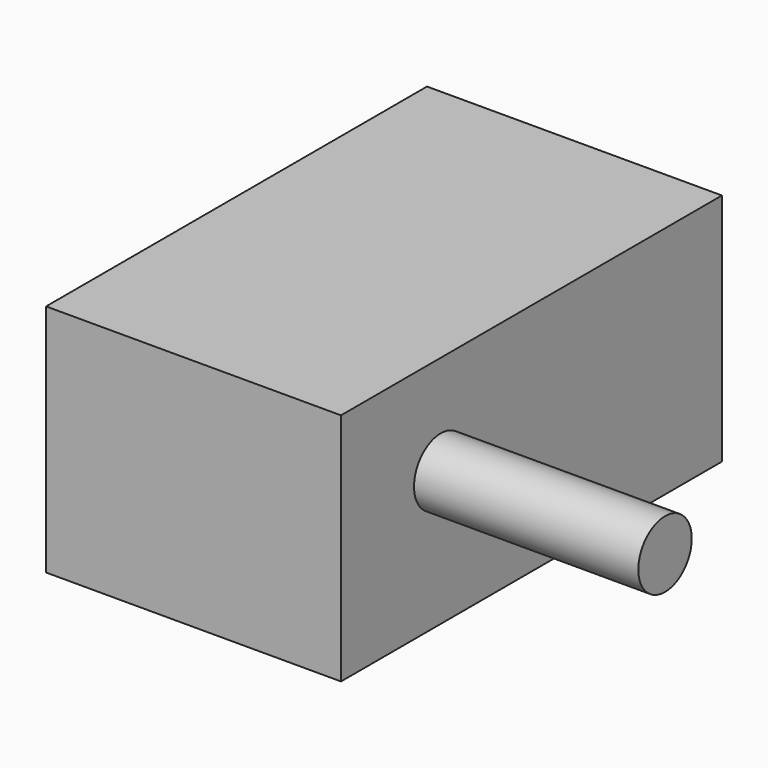
from build123d import *

# Parameters (mm, degrees)
F0_W     = 66.2436261773
F0_H     = 52.6286661625
F1_DEPTH = 53.9066623896
F2_DEPTH = 53.045405075
F3_R     = 7.4993670996
F4_DEPTH = 84.1025914997


# Not quite as in the source:
# - a feature names something its author has since deleted; it is built from what else it names


with BuildPart() as f1:
    # F0 (on Front) → F1 (new body)
    with BuildSketch(Plane.XZ):
        with Locations((0.5984865129, -0.1306533813)):
            Rectangle(F0_W, F0_H)
    extrude(amount=F1_DEPTH)

    # F2 (add): a face of the model
    f2_faces = [f1.faces().sort_by_distance(p)[0] for p in [
        (0.5984865129, 0, -0.1306533813),
    ]]
    extrude(f2_faces, amount=F2_DEPTH)

    # F3 (on Right) → F4 (join)
    with BuildSketch(Plane.YZ):
        with Locations((-25.9069353342, 3.7534534931)):
            Circle(F3_R)
    extrude(amount=F4_DEPTH)


solid = f1.part
